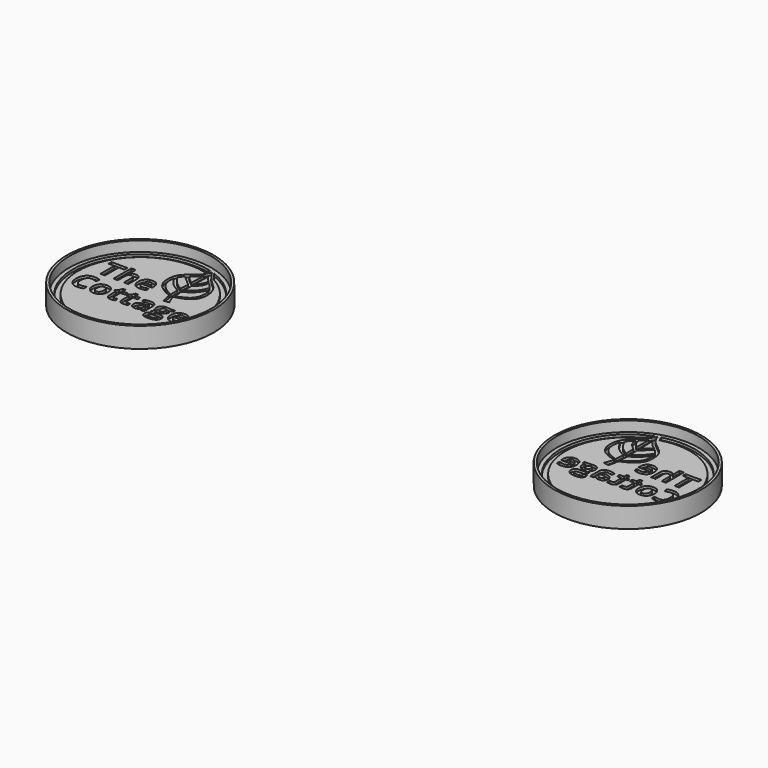
from build123d import *

# Parameters (mm, degrees)
F0_R         = 22.987
F1_DEPTH     = 6.35
F2_R         = 22.225
F3_DEPTH     = 3.175
F4_TEXT_SIZE = 9.1722222222
F5_DEPTH     = 0.762
F7_DEPTH     = 0.762
F9_DEPTH     = 0.762


# Not quite as in the source:
# - Text() gives the source's letters only with a copy of the font that has no kerning and outlines rounded to 1/6400 em; it was checked with that copy


with BuildPart() as f1:
    # F0 (on Top) → F1 (new body)
    with BuildSketch(Plane.XY):
        Circle(F0_R)
    extrude(amount=F1_DEPTH)

    # F2 (on face) → F3 (cut)
    with BuildSketch(Plane.XY.offset(6.35)):
        Circle(F2_R)
    extrude(amount=-F3_DEPTH, mode=Mode.SUBTRACT)

    # F4 (on face) → F5 (cut)
    with BuildSketch(Plane.XY.offset(3.175)):
        with Locations((-16.1874919822, 2.2424466183)):
            Text('The', F4_TEXT_SIZE, font='Open Sans', font_style=FontStyle.BOLD, text_align=(TextAlign.LEFT, TextAlign.BOTTOM))
        with Locations((-17.864008231, -6.604)):
            Text('Cottage', F4_TEXT_SIZE, font='Open Sans', font_style=FontStyle.BOLD, text_align=(TextAlign.LEFT, TextAlign.BOTTOM))
    extrude(amount=-F5_DEPTH, mode=Mode.SUBTRACT)

    # F6 (on face) → F7 (cut)
    with BuildSketch(Plane.XY.offset(3.175)):
        with BuildLine():
            add(Edge.make_bspline(
                [(5.9631960467, 4.3163713999), (5.9772008426, 4.1241503872), (5.9936088662, 3.9410988277), (6.0121374329, 3.7661381454)],
                knots=[0.7211894824, 0.7211894824, 0.7211894824, 0.7211894824, 0.7539851469, 0.7539851469, 0.7539851469, 0.7539851469], degree=3))
            add(Edge.make_bspline(
                [(5.9631960467, 4.3163713999), (4.1538079418, 5.3717940301), (1.2257635687, 7.0797329103), (1.0164149832, 10.28914248), (1.265290838, 11.3985791351)],
                knots=[0, 0, 0, 0, 0.2868027043, 0.4641188047, 0.4641188047, 0.4641188047, 0.4641188047], degree=3))
            add(Edge.make_bspline(
                [(1.265290838, 11.3985791351), (1.3472536205, 11.7639521254), (1.4648841185, 12.1166662696), (1.6157545914, 12.4447244991)],
                knots=[0.4641188047, 0.4641188047, 0.4641188047, 0.4641188047, 0.5225146703, 0.5225146703, 0.5225146703, 0.5225146703], degree=3))
            add(Edge.make_bspline(
                [(1.6157545914, 12.4447244991), (1.6849797456, 12.5952501855), (1.998053202, 13.1921870859), (2.4252288596, 13.6820023244), (2.7756644514, 14.0177160501)],
                knots=[0.5225146703, 0.5225146703, 0.5225146703, 0.5225146703, 0.5493089311, 0.6325673323, 0.6325673323, 0.6325673323, 0.6325673323], degree=3))
            add(Edge.make_bspline(
                [(2.7756644514, 14.0177160501), (3.0385758931, 14.2695825321), (3.3168328772, 14.5018347323), (3.5943708988, 14.7256474417)],
                knots=[0.6325673323, 0.6325673323, 0.6325673323, 0.6325673323, 0.695031268, 0.695031268, 0.695031268, 0.695031268], degree=3))
            add(Edge.make_bspline(
                [(3.5943708988, 14.7256474417), (4.0265618755, 15.0741756646), (5.3761242642, 16.1027356582), (6.1122381895, 17.3449288826), (6.6135660745, 18.1909203529)],
                knots=[0.695031268, 0.695031268, 0.695031268, 0.695031268, 0.7923020824, 1, 1, 1, 1], degree=3))
            add(Edge.make_bspline(
                [(6.6135660745, 18.1909203529), (7.2150157041, 17.4014303779), (7.8850180247, 16.5219550414), (8.8716548457, 15.5550968025), (8.975028396, 15.4550258323)],
                knots=[0, 0, 0, 0, 0.2098911941, 0.2338144048, 0.2338144048, 0.2338144048, 0.2338144048], degree=3))
            add(Edge.make_bspline(
                [(8.975028396, 15.4550258323), (9.1619707391, 15.2740559266), (9.356839592, 15.0893419608), (9.5543651671, 14.8995233715)],
                knots=[0.2338144048, 0.2338144048, 0.2338144048, 0.2338144048, 0.2770775126, 0.2770775126, 0.2770775126, 0.2770775126], degree=3))
            add(Edge.make_bspline(
                [(9.5543651671, 14.8995233715), (10.1442418685, 14.3326622788), (10.7578116736, 13.7202772789), (11.254726386, 13.0261330195)],
                knots=[0.2770775126, 0.2770775126, 0.2770775126, 0.2770775126, 0.4062754624, 0.4062754624, 0.4062754624, 0.4062754624], degree=3))
            add(Edge.make_bspline(
                [(11.254726386, 13.0261330195), (11.5177420058, 12.6587243313), (11.7480760434, 12.2684103254), (11.9249168783, 11.8498178199)],
                knots=[0.4062754624, 0.4062754624, 0.4062754624, 0.4062754624, 0.4746595895, 0.4746595895, 0.4746595895, 0.4746595895], degree=3))
            add(Edge.make_bspline(
                [(11.9249168783, 11.8498178199), (12.6003183726, 10.251103339), (12.3893365992, 6.2056923438), (8.9788655623, 4.9485274106), (7.2639356367, 4.3163713999)],
                knots=[0.4746595895, 0.4746595895, 0.4746595895, 0.4746595895, 0.7358364926, 1, 1, 1, 1], degree=3))
            add(Edge.make_bspline(
                [(7.3374421612, 3.819138692), (7.3104673277, 3.9772422892), (7.2858666201, 4.1426820538), (7.2639356367, 4.3163713999)],
                knots=[0.2441251643, 0.2441251643, 0.2441251643, 0.2441251643, 0.2745207852, 0.2745207852, 0.2745207852, 0.2745207852], degree=3))
            add(Edge.make_bspline(
                [(7.3374421612, 3.819138692), (8.3690525015, 4.1042087718), (10.3853785815, 4.6613903102), (12.8010967273, 6.5850148923), (13.4623430297, 9.6750633165), (12.726733863, 12.909458673), (10.8352244135, 14.9008201383), (8.6503105225, 16.7052736459), (7.2875874376, 18.7233226397), (6.5557751805, 19.8070593178)],
                knots=[0, 0, 0, 0, 0.145369021, 0.2841299053, 0.4256285973, 0.5718175889, 0.7048599145, 0.8415032852, 1, 1, 1, 1], degree=3))
            add(Edge.make_bspline(
                [(6.0121374329, 3.7661381454), (4.9410027831, 4.2422042179), (2.8645918291, 5.1650656042), (0.612888038, 7.491981372), (0.1831525135, 10.371019873), (0.5977945397, 13.5657239381), (3.3730529116, 15.8009371387), (5.5774022203, 17.472984829), (6.2361237446, 19.0444766503), (6.5557751805, 19.8070593178)],
                knots=[0, 0, 0, 0, 0.1537920739, 0.298128295, 0.4363785907, 0.5805841433, 0.7337052222, 0.8707777036, 1, 1, 1, 1], degree=3))
        make_face()
        with BuildLine():
            add(Edge.make_bspline(
                [(5.8957659448, 7.1296877589), (5.8878881246, 6.0963594858), (5.9042671992, 5.1251916634), (5.9631960467, 4.3163713999)],
                knots=[0.5831931332, 0.5831931332, 0.5831931332, 0.5831931332, 0.7211894824, 0.7211894824, 0.7211894824, 0.7211894824], degree=3))
            add(Edge.make_bspline(
                [(5.9631960467, 4.3163713999), (5.9772008426, 4.1241503872), (5.9936088662, 3.9410988277), (6.0121374329, 3.7661381454)],
                knots=[0.7211894824, 0.7211894824, 0.7211894824, 0.7211894824, 0.7539851469, 0.7539851469, 0.7539851469, 0.7539851469], degree=3))
            add(Edge.make_bspline(
                [(6.0121374329, 3.7661381454), (6.4555079614, 3.7841187735), (6.8940716327, 3.8011580639), (7.3374421612, 3.819138692)],
                knots=[0, 0, 0, 0, 1.326364083, 1.326364083, 1.326364083, 1.326364083], degree=3))
            add(Edge.make_bspline(
                [(7.3374421612, 3.819138692), (7.3104673277, 3.9772422892), (7.2858666201, 4.1426820538), (7.2639356367, 4.3163713999)],
                knots=[0.2441251643, 0.2441251643, 0.2441251643, 0.2441251643, 0.2745207852, 0.2745207852, 0.2745207852, 0.2745207852], degree=3))
            add(Edge.make_bspline(
                [(7.2639356367, 4.3163713999), (7.1630845628, 5.1150933177), (7.1186896388, 6.0882675592), (7.1072613151, 7.1296877589)],
                knots=[0.2745207852, 0.2745207852, 0.2745207852, 0.2745207852, 0.4142970533, 0.4142970533, 0.4142970533, 0.4142970533], degree=3))
            add(Edge.make_bspline(
                [(7.1072613151, 7.1296877589), (7.1035331476, 7.4694216609), (7.1033133061, 7.81641834), (7.1057863105, 8.1669906597)],
                knots=[0.4142970533, 0.4142970533, 0.4142970533, 0.4142970533, 0.4598951097, 0.4598951097, 0.4598951097, 0.4598951097], degree=3))
            add(Edge.make_bspline(
                [(7.1057863105, 8.1669906597), (7.1127900737, 9.1598419228), (7.1413923895, 10.1813723837), (7.1730693305, 11.147827392)],
                knots=[0.4598951097, 0.4598951097, 0.4598951097, 0.4598951097, 0.5890327663, 0.5890327663, 0.5890327663, 0.5890327663], degree=3))
            add(Edge.make_bspline(
                [(7.1730693305, 11.147827392), (7.1869814771, 11.572283268), (7.2014866773, 11.9861158331), (7.2150157041, 12.382229936)],
                knots=[0.5890327663, 0.5890327663, 0.5890327663, 0.5890327663, 0.6457485334, 0.6457485334, 0.6457485334, 0.6457485334], degree=3))
            add(Edge.make_bspline(
                [(7.2150157041, 12.382229936), (7.2352612434, 12.9749956806), (7.3106404269, 15.2835439333), (7.2563210859, 16.4866030645), (7.2150157041, 17.4014303779)],
                knots=[0.6457485334, 0.6457485334, 0.6457485334, 0.6457485334, 0.730620957, 1, 1, 1, 1], degree=3))
            add(Edge.make_bspline(
                [(7.2150157041, 17.4014303779), (7.5618411993, 16.9729661971), (8.192436151, 16.193936532), (8.7321539206, 15.6843439092), (8.975028396, 15.4550258323)],
                knots=[0, 0, 0, 0, 0.5499972594, 1, 1, 1, 1], degree=3))
            add(Edge.make_bspline(
                [(6.6135660745, 18.1909203529), (7.2150157041, 17.4014303779), (7.8850180247, 16.5219550414), (8.8716548457, 15.5550968025), (8.975028396, 15.4550258323)],
                knots=[0, 0, 0, 0, 0.2098911941, 0.2338144048, 0.2338144048, 0.2338144048, 0.2338144048], degree=3))
            add(Edge.make_bspline(
                [(3.5943708988, 14.7256474417), (4.0265618755, 15.0741756646), (5.3761242642, 16.1027356582), (6.1122381895, 17.3449288826), (6.6135660745, 18.1909203529)],
                knots=[0.695031268, 0.695031268, 0.695031268, 0.695031268, 0.7923020824, 1, 1, 1, 1], degree=3))
            add(Edge.make_bspline(
                [(6.1122381895, 17.3449288826), (5.76756141, 16.822361347), (5.0826647739, 15.7839834563), (4.0883119606, 15.0768923292), (3.5943708988, 14.7256474417)],
                knots=[0, 0, 0, 0, 0.5032537193, 1, 1, 1, 1], degree=3))
            add(Edge.make_bspline(
                [(6.1342608543, 16.2403699158), (6.1335159351, 16.6986367116), (6.1228770623, 17.0217827971), (6.1122381895, 17.3449288826)],
                knots=[0.6602579057, 0.6602579057, 0.6602579057, 0.6602579057, 1, 1, 1, 1], degree=3))
            add(Edge.make_bspline(
                [(6.1342608543, 16.2403699158), (6.1413692648, 15.6361871671), (6.1376657682, 14.5869101912), (6.0786802213, 13.0146209942), (6.0563124664, 12.4447244991)],
                knots=[0.1051017626, 0.1051017626, 0.1051017626, 0.1051017626, 0.2663516079, 0.3486787638, 0.3486787638, 0.3486787638, 0.3486787638], degree=3))
            add(Edge.make_bspline(
                [(6.0563124664, 12.4447244991), (6.0405275532, 12.0425488339), (6.0235319271, 11.6212122552), (6.0066906992, 11.1881912538)],
                knots=[0.3486787638, 0.3486787638, 0.3486787638, 0.3486787638, 0.4067769957, 0.4067769957, 0.4067769957, 0.4067769957], degree=3))
            add(Edge.make_bspline(
                [(6.0066906992, 11.1881912538), (5.9700449403, 10.2459569171), (5.934130223, 9.2483993927), (5.9130108399, 8.2725465163)],
                knots=[0.4067769957, 0.4067769957, 0.4067769957, 0.4067769957, 0.5331961503, 0.5331961503, 0.5331961503, 0.5331961503], degree=3))
            add(Edge.make_bspline(
                [(5.9130108399, 8.2725465163), (5.9046584234, 7.886610543), (5.8986201308, 7.5040693727), (5.8957659448, 7.1296877589)],
                knots=[0.5331961503, 0.5331961503, 0.5331961503, 0.5331961503, 0.5831931332, 0.5831931332, 0.5831931332, 0.5831931332], degree=3))
        make_face()
        with BuildLine():
            add(Edge.make_bspline(
                [(1.265290838, 11.3985791351), (1.3472536205, 11.7639521254), (1.4648841185, 12.1166662696), (1.6157545914, 12.4447244991)],
                knots=[0.4641188047, 0.4641188047, 0.4641188047, 0.4641188047, 0.5225146703, 0.5225146703, 0.5225146703, 0.5225146703], degree=3))
            add(Edge.make_bspline(
                [(5.8957659448, 7.1296877589), (4.9942717271, 7.6647057881), (3.1755769963, 8.7450081045), (1.9043927584, 10.5088241273), (1.265290838, 11.3985791351)],
                knots=[0, 0, 0, 0, 0.4954912023, 1, 1, 1, 1], degree=3))
            add(Edge.make_bspline(
                [(5.9130108399, 8.2725465163), (5.9046584234, 7.886610543), (5.8986201308, 7.5040693727), (5.8957659448, 7.1296877589)],
                knots=[0.5331961503, 0.5331961503, 0.5331961503, 0.5331961503, 0.5831931332, 0.5831931332, 0.5831931332, 0.5831931332], degree=3))
            add(Edge.make_bspline(
                [(5.9130108399, 8.2725465163), (5.1598743814, 8.7363339777), (3.5771755081, 9.7202821367), (2.292356036, 11.5028942432), (1.6157545914, 12.4447244991)],
                knots=[0, 0, 0, 0, 0.4725147068, 1, 1, 1, 1], degree=3))
        make_face()
        with BuildLine():
            add(Edge.make_bspline(
                [(6.0121374329, 3.7661381454), (6.4555079614, 3.7841187735), (6.8940716327, 3.8011580639), (7.3374421612, 3.819138692)],
                knots=[0, 0, 0, 0, 1.326364083, 1.326364083, 1.326364083, 1.326364083], degree=3))
            add(Edge.make_bspline(
                [(6.0121374329, 3.7661381454), (6.1511284454, 2.4536803188), (6.4094459529, 1.5965096506), (6.6677634604, 0.7393389824)],
                knots=[0.7539851469, 0.7539851469, 0.7539851469, 0.7539851469, 1, 1, 1, 1], degree=3))
            add(Edge.make_bspline(
                [(8.2936873659, 0.9561289335), (7.7517127308, 0.8838656164), (7.2097380956, 0.8116022994), (6.6677634604, 0.7393389824)],
                knots=[0, 0, 0, 0, 1.640312906, 1.640312906, 1.640312906, 1.640312906], degree=3))
            add(Edge.make_bspline(
                [(8.2936873659, 0.9561289335), (7.9238901647, 1.7527221783), (7.5540929635, 2.5493154232), (7.3374421612, 3.819138692)],
                knots=[0, 0, 0, 0, 0.2441251643, 0.2441251643, 0.2441251643, 0.2441251643], degree=3))
        make_face()
        with BuildLine():
            add(Edge.make_bspline(
                [(2.7756644514, 14.0177160501), (3.0385758931, 14.2695825321), (3.3168328772, 14.5018347323), (3.5943708988, 14.7256474417)],
                knots=[0.6325673323, 0.6325673323, 0.6325673323, 0.6325673323, 0.695031268, 0.695031268, 0.695031268, 0.695031268], degree=3))
            add(Edge.make_bspline(
                [(6.006690708, 11.1881912592), (5.5084205843, 11.593520091), (4.4568295059, 12.4509193427), (3.3550259183, 13.4777680919), (2.7756644514, 14.0177160501)],
                knots=[0.0154968755, 0.0154968755, 0.0154968755, 0.0154968755, 0.4823186449, 1, 1, 1, 1], degree=3))
            add(Edge.make_bspline(
                [(6.0563124664, 12.4447244991), (6.0405275532, 12.0425488339), (6.0235319271, 11.6212122552), (6.0066906992, 11.1881912538)],
                knots=[0.3486787638, 0.3486787638, 0.3486787638, 0.3486787638, 0.4067769957, 0.4067769957, 0.4067769957, 0.4067769957], degree=3))
            add(Edge.make_bspline(
                [(6.0563124664, 12.4447244991), (5.2995949392, 13.0088282974), (4.0976568683, 13.9088851738), (3.7306849713, 14.5038999939), (3.5943708988, 14.7256474417)],
                knots=[0, 0, 0, 0, 0.6270968623, 1, 1, 1, 1], degree=3))
        make_face()
        with BuildLine():
            add(Edge.make_bspline(
                [(6.0563124664, 12.4447244991), (6.0946875749, 13.8473549294), (6.1344528191, 15.300795552), (6.1343114632, 16.2092358252), (6.1342608543, 16.2403699158)],
                knots=[0, 0, 0, 0, 0.6371762397, 0.6602579057, 0.6602579057, 0.6602579057, 0.6602579057], degree=3))
            add(Edge.make_bspline(
                [(6.1342608543, 16.2403699158), (6.1413692648, 15.6361871671), (6.1376657682, 14.5869101912), (6.0786802213, 13.0146209942), (6.0563124664, 12.4447244991)],
                knots=[0.1051017626, 0.1051017626, 0.1051017626, 0.1051017626, 0.2663516079, 0.3486787638, 0.3486787638, 0.3486787638, 0.3486787638], degree=3))
        make_face()
        with BuildLine():
            add(Edge.make_bspline(
                [(7.1072613151, 7.1296877589), (7.1035331476, 7.4694216609), (7.1033133061, 7.81641834), (7.1057863105, 8.1669906597)],
                knots=[0.4142970533, 0.4142970533, 0.4142970533, 0.4142970533, 0.4598951097, 0.4598951097, 0.4598951097, 0.4598951097], degree=3))
            add(Edge.make_bspline(
                [(7.1072613151, 7.1296877589), (7.9907071257, 7.587310128), (9.8870450707, 8.5568258408), (11.2179361954, 10.710854651), (11.9249168783, 11.8498178199)],
                knots=[0, 0, 0, 0, 0.4700816547, 1, 1, 1, 1], degree=3))
            add(Edge.make_bspline(
                [(11.254726386, 13.0261330195), (11.5177420058, 12.6587243313), (11.7480760434, 12.2684103254), (11.9249168783, 11.8498178199)],
                knots=[0.4062754624, 0.4062754624, 0.4062754624, 0.4062754624, 0.4746595895, 0.4746595895, 0.4746595895, 0.4746595895], degree=3))
            add(Edge.make_bspline(
                [(7.1057863105, 8.1669906597), (8.131076101, 8.8493337812), (10.1032375863, 10.1569504725), (10.8897083673, 12.1025499883), (11.254726386, 13.0261330195)],
                knots=[0, 0, 0, 0, 0.521439433, 1, 1, 1, 1], degree=3))
        make_face()
        with BuildLine():
            add(Edge.make_bspline(
                [(8.975028396, 15.4550258323), (9.1619707391, 15.2740559266), (9.356839592, 15.0893419608), (9.5543651671, 14.8995233715)],
                knots=[0.2338144048, 0.2338144048, 0.2338144048, 0.2338144048, 0.2770775126, 0.2770775126, 0.2770775126, 0.2770775126], degree=3))
            add(Edge.make_bspline(
                [(7.2150157041, 12.382229936), (7.611314005, 12.7447925822), (8.447892041, 13.5099088941), (8.7925406857, 14.783805622), (8.975028396, 15.4550258323)],
                knots=[0, 0, 0, 0, 0.473852604, 1, 1, 1, 1], degree=3))
            add(Edge.make_bspline(
                [(7.1730693305, 11.147827392), (7.1869814771, 11.572283268), (7.2014866773, 11.9861158331), (7.2150157041, 12.382229936)],
                knots=[0.5890327663, 0.5890327663, 0.5890327663, 0.5890327663, 0.6457485334, 0.6457485334, 0.6457485334, 0.6457485334], degree=3))
            add(Edge.make_bspline(
                [(9.5543651671, 14.8995233715), (9.4673762878, 14.2844949467), (9.2752743076, 12.9303541897), (7.9163635129, 11.7771729032), (7.1730693305, 11.147827392)],
                knots=[0, 0, 0, 0, 0.4539986314, 1, 1, 1, 1], degree=3))
        make_face()
    extrude(amount=-F7_DEPTH, mode=Mode.SUBTRACT)

    # F8 (on face) → F9 (cut)
    with BuildSketch(Plane.XY.offset(3.175)):
        with BuildLine():
            ThreePointArc((9.2397885219, 17.1386166853), (-7.2053756192, -18.088350837), (5.0751554975, 18.7975708668))
            add(Edge.make_bspline(
                [(5.0751554975, 18.7975708668), (5.2067168765, 19.0229672579), (5.4705269261, 19.4742299484), (5.6429345728, 19.9694803047), (5.7277825101, 20.2112406209)],
                knots=[0, 0, 0, 0, 0.5009376302, 1, 1, 1, 1], degree=3))
            ThreePointArc((5.7277825101, 20.2112406209), (-6.5379273455, -19.9638985658), (7.3374421612, 19.6840971967))
            add(Edge.make_bspline(
                [(9.2397885219, 17.1386166853), (8.8774015228, 17.6840518728), (8.1991692661, 18.667318531), (7.6086264104, 19.3671516614), (7.3374421612, 19.6840971967)],
                knots=[0, 0, 0, 0, 0.5447351422, 1, 1, 1, 1], degree=3))
        make_face()
    extrude(amount=-F9_DEPTH, mode=Mode.SUBTRACT)


with BuildPart() as f11_1:
    # F11: instance of F1
    add(f1.part.mirror(Plane.YZ.offset(76.2)))


solid = Compound([f1.part, f11_1.part])
